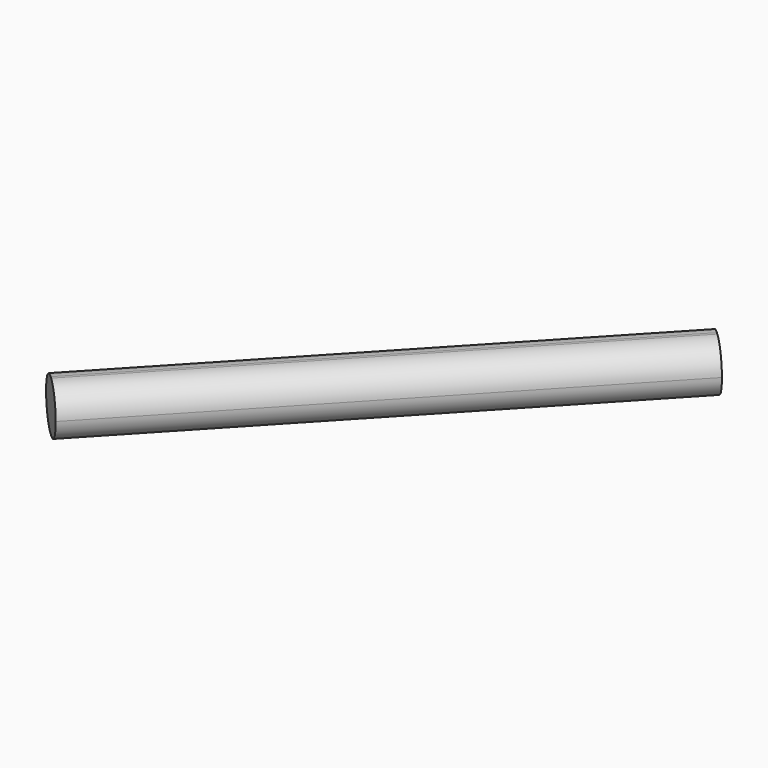
from build123d import *

# Parameters (mm, degrees)
F1_DEPTH = 50.8
F2_R     = 25.39999


# Not quite as in the source:
# - a fillet or chamfer is up to 0.001 mm smaller than in the source, because OpenCascade refuses the exact size


with BuildPart() as f1:
    # F0 (on Top) → F1 (new body)
    with BuildSketch(Plane.XY):
        Polygon((-38.8906911175, 36.5057453632), (0, 0), (362.7456650138, 386.4440917969), (323.8549738963, 422.9498371601), align=None)
    extrude(amount=F1_DEPTH)

    # F2 (radius 25.4 in the source; OpenCascade refuses exactly that, so slightly less here)
    f2_edges = [f1.edges().sort_by_distance(p)[0] for p in [
        (142.482141, 229.727791, 50.8),
        (181.372833, 193.222046, 50.8),
        (181.372833, 193.222046, 0),
        (142.482141, 229.727791, 0),
    ]]
    fillet(f2_edges, radius=F2_R)


solid = f1.part
